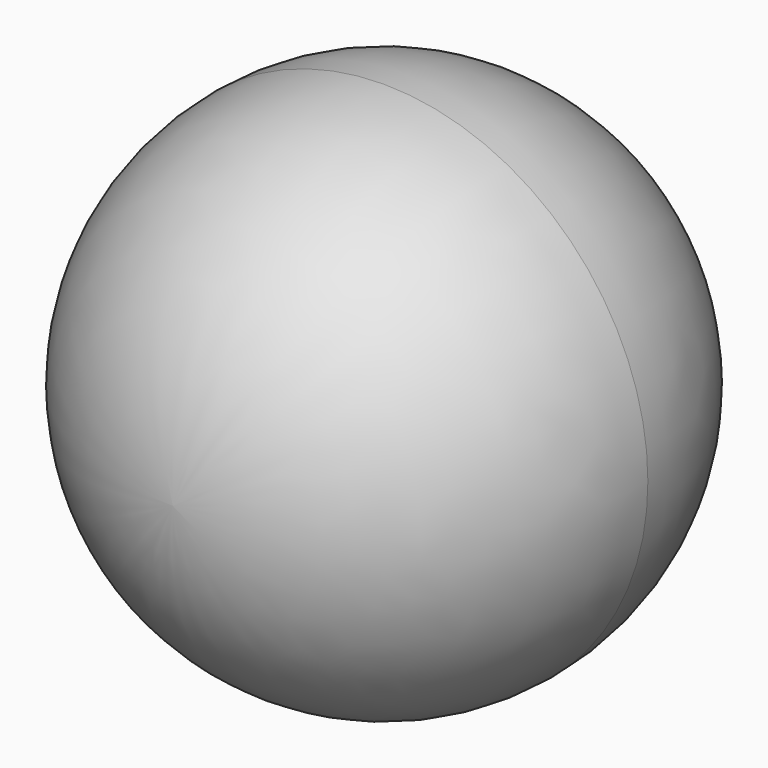
from build123d import *

# Parameters (mm, degrees)
F0_R     = 30
F1_DEPTH = 60
F2_R     = 29.99999


# Not quite as in the source:
# - a fillet or chamfer is up to 0.001 mm smaller than in the source, because OpenCascade refuses the exact size


with BuildPart() as f1:
    # F0 (on Front) → F1 (new body)
    with BuildSketch(Plane.XZ):
        Circle(F0_R)
    extrude(amount=F1_DEPTH)

    # F2 (radius 30 in the source; OpenCascade refuses exactly that, so slightly less here)
    f2_edges = [f1.edges().sort_by_distance(p)[0] for p in [
        (30, -30, 0),
        (-30, 0, 0),
        (-30, -60, 0),
    ]]
    fillet(f2_edges, radius=F2_R)


solid = f1.part
